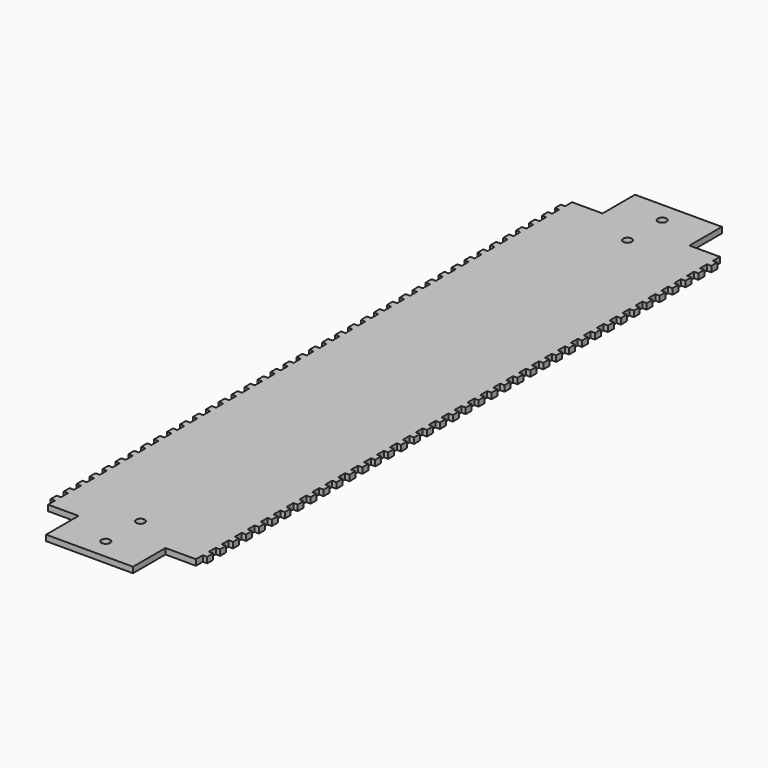
from build123d import *
from build123d import SkipClean  # not in build123d's __all__

# Parameters (mm, degrees)
F1_DEPTH         = 1
F4_W             = 0.75
F4_H             = 0.75
F5_DEPTH         = 1
F5_COPIES_COUNT  = 6
F5_COPIES_PITCH  = 11.15
F5_COPIES2_COUNT = 2


# Not quite as in the source:
# - a pattern or mirror of a feature is missing from the dataset's text; its kind, count and spacing are read off the source's solid


with BuildPart() as f1:
    # F0 (on Top) → F1 (new body)
    with BuildSketch(Plane.XY):
        with BuildLine():
            Line((-13.5, 56.5), (-13.5, 0))
            Line((-13.5, 0), (0, 0))
            Line((0, 0), (0, 51.75))
            ThreePointArc((0, 51.75), (-0.75, 52.5), (0, 53.25))
            Line((0, 53.25), (0, 59.25))
            ThreePointArc((0, 59.25), (-0.75, 60), (0, 60.75))
            Line((0, 60.75), (0, 63.5))
            Line((0, 63.5), (-7.5, 63.5))
            Line((-7.5, 63.5), (-7.5, 56.5))
            Line((-7.5, 56.5), (-13.5, 56.5))
        make_face()
    extrude(amount=F1_DEPTH)

    # F2: F1 across face


with BuildPart() as f1_1:
    add(f1.part, clean=False)
    with SkipClean():  # cleaning this boolean's faces spoils the solid; the shape is the same uncleaned
        add(f1.part.mirror(Plane(origin=(0, 25.875, 0.5), x_dir=(0, 1, 0), z_dir=(1, 0, 0))), clean=False)

    # F3: F1 across face


with BuildPart() as f1_2:
    add(f1_1.part, clean=False)
    add(f1_1.part.mirror(Plane(origin=(-6.75, 0, 0.5), x_dir=(1, 0, 0), z_dir=(0, -1, 0))), clean=False)

    # F4 (on face) → F5 (cut, through all)
    with BuildSketch(Plane.XY.offset(1)):
        Polygon((-13.5, 53.7125), (-13.5, 55), (-13.5, 56.5), (-14.5, 56.5), (-14.5, 0), (-13.5, 0), (-13.5, 0.75), (-13.5, 2.0375), (-13.5, 3.5375), (-13.5, 4.825), (-13.5, 6.325), (-13.5, 7.6125), (-13.5, 9.1125), (-13.5, 10.4), (-13.5, 11.9), (-13.5, 13.1875), (-13.5, 14.6875), (-13.5, 15.975), (-13.5, 17.475), (-13.5, 18.7625), (-13.5, 20.2625), (-13.5, 21.55), (-13.5, 23.05), (-13.5, 24.3375), (-13.5, 25.8375), (-13.5, 27.125), (-13.5, 28.625), (-13.5, 29.9125), (-13.5, 31.4125), (-13.5, 32.7), (-13.5, 34.2), (-13.5, 35.4875), (-13.5, 36.9875), (-13.5, 38.275), (-13.5, 39.775), (-13.5, 41.0625), (-13.5, 42.5625), (-13.5, 43.85), (-13.5, 45.35), (-13.5, 46.6375), (-13.5, 48.1375), (-13.5, 49.425), (-13.5, 50.925), (-13.5, 52.2125), align=None)
        Polygon((-12.75, 50.925), (-13.5, 50.925), (-13.5, 49.425), (-12.75, 49.425), (-12.75, 50.175), align=None)
        Polygon((-12.75, 55), (-12.75, 55.75), (-12.75, 56.5), (-13.5, 56.5), (-13.5, 55), align=None)
        Polygon((-12.75, 53.7125), (-13.5, 53.7125), (-13.5, 52.2125), (-12.75, 52.2125), (-12.75, 52.9625), align=None)
        Polygon((-12.75, 48.1375), (-13.5, 48.1375), (-13.5, 46.6375), (-12.75, 46.6375), (-12.75, 47.3875), align=None)
        Polygon((-12.75, 45.35), (-13.5, 45.35), (-13.5, 43.85), (-12.75, 43.85), (-12.75, 44.6), align=None)
        Polygon((-12.75, 42.5625), (-13.5, 42.5625), (-13.5, 41.0625), (-12.75, 41.0625), (-12.75, 41.8125), align=None)
        Polygon((-12.75, 39.775), (-13.5, 39.775), (-13.5, 38.275), (-12.75, 38.275), (-12.75, 39.025), align=None)
        Polygon((-12.75, 36.9875), (-13.5, 36.9875), (-13.5, 35.4875), (-12.75, 35.4875), (-12.75, 36.2375), align=None)
        Polygon((-12.75, 34.2), (-13.5, 34.2), (-13.5, 32.7), (-12.75, 32.7), (-12.75, 33.45), align=None)
        Polygon((-12.75, 31.4125), (-13.5, 31.4125), (-13.5, 29.9125), (-12.75, 29.9125), (-12.75, 30.6625), align=None)
        Polygon((-12.75, 28.625), (-13.5, 28.625), (-13.5, 27.125), (-12.75, 27.125), (-12.75, 27.875), align=None)
        Polygon((-12.75, 25.8375), (-13.5, 25.8375), (-13.5, 24.3375), (-12.75, 24.3375), (-12.75, 25.0875), align=None)
        Polygon((-13.5, 23.05), (-13.5, 21.55), (-12.75, 21.55), (-12.75, 22.3), (-12.75, 23.05), align=None)
        Polygon((-13.5, 20.2625), (-13.5, 18.7625), (-12.75, 18.7625), (-12.75, 19.5125), (-12.75, 20.2625), align=None)
        Polygon((-13.5, 17.475), (-13.5, 15.975), (-12.75, 15.975), (-12.75, 16.725), (-12.75, 17.475), align=None)
        Polygon((-13.5, 14.6875), (-13.5, 13.1875), (-12.75, 13.1875), (-12.75, 13.9375), (-12.75, 14.6875), align=None)
        Polygon((-13.5, 11.9), (-13.5, 10.4), (-12.75, 10.4), (-12.75, 11.15), (-12.75, 11.9), align=None)
        Polygon((-13.5, 9.1125), (-13.5, 7.6125), (-12.75, 7.6125), (-12.75, 8.3625), (-12.75, 9.1125), align=None)
        Polygon((-13.5, 6.325), (-13.5, 4.825), (-12.75, 4.825), (-12.75, 5.575), (-12.75, 6.325), align=None)
        Polygon((-13.5, 3.5375), (-13.5, 2.0375), (-12.75, 2.0375), (-12.75, 2.7875), (-12.75, 3.5375), align=None)
        with Locations((-13.125, 0.375)):
            Rectangle(F4_W, F4_H)
    f5 = extrude(amount=-F5_DEPTH, mode=Mode.SUBTRACT)

    # F5_copies: F5 ×6
    with Locations(*[(0, -i * F5_COPIES_PITCH, 0) for i in range(1, F5_COPIES_COUNT)]):
        add(f5, clean=False, mode=Mode.SUBTRACT)

    # F5_copies1: F5 across plane
    add(f5.mirror(Plane(origin=(0, 0, 0), x_dir=(0, 0, 1), z_dir=(1, 0, 0))), clean=False, mode=Mode.SUBTRACT)

    # F5_copies2: F5 ×2 about axis
    f5_copies2_axis = Axis((0, 0, 0), (0, 0, 1))
    for i in range(1, F5_COPIES2_COUNT):
        add(f5.rotate(f5_copies2_axis, i * 360 / F5_COPIES2_COUNT), clean=False, mode=Mode.SUBTRACT)

    # F5_copies3: F5 across plane
    add(f5.mirror(Plane(origin=(0, -19.5125, 0), x_dir=(0, 0, -1), z_dir=(0, -1, 0))), clean=False, mode=Mode.SUBTRACT)


solid = f1_2.part
